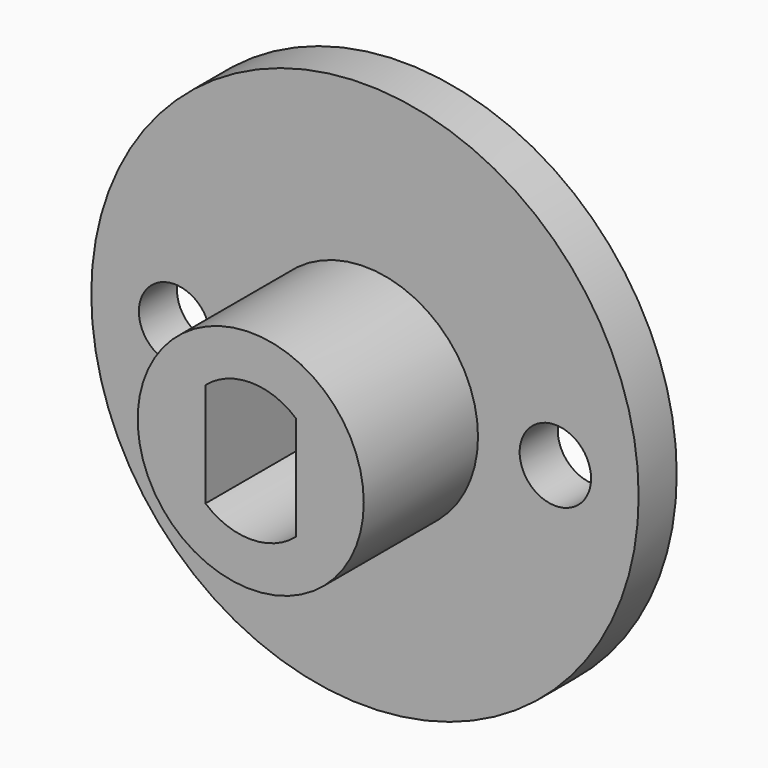
from build123d import *

# Parameters (mm, degrees)
F0_R     = 4.75
F1_DEPTH = 8
F0_R_2   = 11.5
F0_R_3   = 1.5
F2_DEPTH = 2


# Not quite as in the source:
# - a feature names something its author has since deleted; it is built from what else it names


with BuildPart() as f1:
    # F0 (on Front) → F1 (new body)
    with BuildSketch(Plane.XZ):
        Circle(F0_R)
        with BuildLine():
            ThreePointArc((1.9, 2.19089023), (2.6381811917, 1.2041594579), (2.9, 0))
            ThreePointArc((2.9, 0), (2.6381811917, -1.2041594579), (1.9, -2.19089023))
            ThreePointArc((1.9, -2.19089023), (0, -2.9), (-1.9, -2.19089023))
            ThreePointArc((-1.9, -2.19089023), (-2.9, 0), (-1.9, 2.19089023))
            ThreePointArc((-1.9, 2.19089023), (0, 2.9), (1.9, 2.19089023))
        make_face(mode=Mode.SUBTRACT)
        with BuildLine():
            Line((-1.9, -2.19089023), (-1.9, 2.19089023))
            ThreePointArc((-1.9, 2.19089023), (-2.9, 0), (-1.9, -2.19089023))
        make_face()
        with BuildLine():
            ThreePointArc((1.9, -2.19089023), (2.6381811917, -1.2041594579), (2.9, 0))
            ThreePointArc((2.9, 0), (2.6381811917, 1.2041594579), (1.9, 2.19089023))
            Line((1.9, 2.19089023), (1.9, -2.19089023))
        make_face()
    extrude(amount=F1_DEPTH)

    # F0 (on Front) → F2 (join)
    with BuildSketch(Plane.XZ):
        Circle(F0_R_2)
        with Locations((-8, 0)):
            Circle(F0_R_3, mode=Mode.SUBTRACT)
        Circle(F0_R, mode=Mode.SUBTRACT)
        with Locations((8, 0)):
            Circle(F0_R_3, mode=Mode.SUBTRACT)
    extrude(amount=F2_DEPTH)


solid = f1.part
